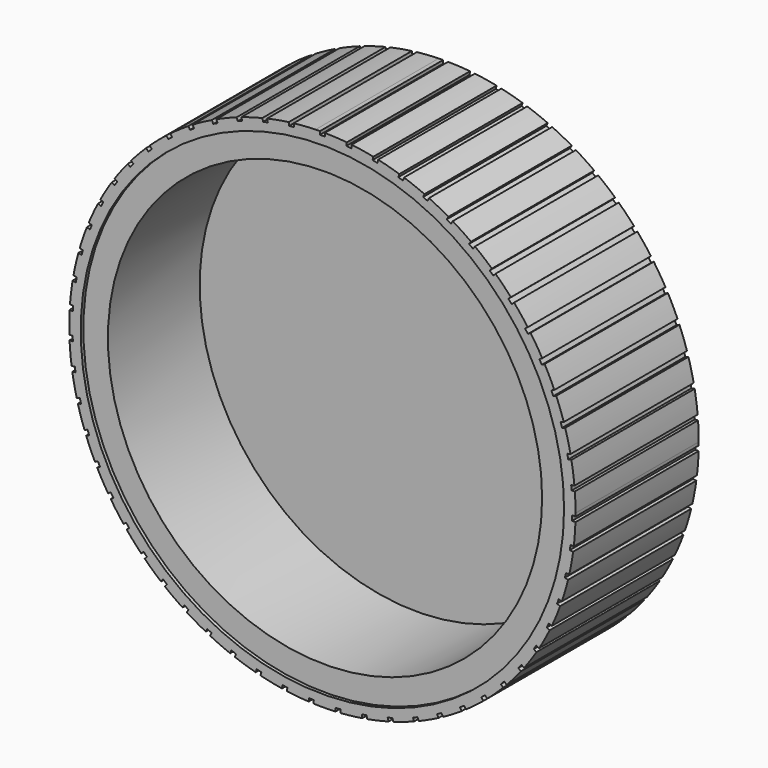
from build123d import *

# Parameters (mm, degrees)
F0_R     = 14.75
F0_R_2   = 13.25
F1_DEPTH = 9
F2_R     = 13.25
F3_DEPTH = 2
F4_R     = 14.75
F5_DEPTH = 9.2
F6_DEPTH = 0.2


# Not quite as in the source:
# - a feature names something its author has since deleted; it is built from what else it names


with BuildPart() as f1:
    # F0 (on Front) → F1 (new body)
    with BuildSketch(Plane.XZ):
        Circle(F0_R)
        Circle(F0_R_2, mode=Mode.SUBTRACT)
    extrude(amount=F1_DEPTH)

    # F2 (on Front) → F3 (join)
    with BuildSketch(Plane.XZ):
        Circle(F2_R)
    extrude(amount=F3_DEPTH)

    # F4 (on Front) → F5 (join)
    with BuildSketch(Plane.XZ):
        with BuildLine():
            ThreePointArc((15.4487973261, -0.1927723482), (15.4496993286, -0.0963880499), (15.45, 0))
            ThreePointArc((15.45, 0), (15.4393387559, 0.5738630326), (15.4073697372, 1.146934079))
            Line((15.4073697372, 1.146934079), (15.2080751315, 1.1301513458))
            Line((15.2080751315, 1.1301513458), (15.1829010317, 1.4290932544))
            Line((15.1829010317, 1.4290932544), (15.3821956374, 1.4458759876))
            ThreePointArc((15.3821956374, 1.4458759876), (15.3049999381, 2.1117473558), (15.1989934484, 2.77364348))
            Line((15.1989934484, 2.77364348), (15.0026005872, 2.7358302011))
            Line((15.0026005872, 2.7358302011), (14.9458806688, 3.0304194929))
            Line((14.9458806688, 3.0304194929), (15.14227353, 3.0682327718))
            ThreePointArc((15.14227353, 3.0682327718), (14.9949308113, 3.7221700611), (14.8193609898, 4.3691005774))
            Line((14.8193609898, 4.3691005774), (14.6280827491, 4.3106828175))
            Line((14.6280827491, 4.3106828175), (14.5404561094, 4.5976001784))
            Line((14.5404561094, 4.5976001784), (14.73173435, 4.6560179383))
            ThreePointArc((14.73173435, 4.6560179383), (14.5159048106, 5.2906528452), (14.2727499076, 5.9153283995))
            Line((14.2727499076, 5.9153283995), (14.0887415342, 5.8369643867))
            Line((14.0887415342, 5.8369643867), (13.9711955149, 6.1129769468))
            Line((13.9711955149, 6.1129769468), (14.1552038884, 6.1913409597))
            ThreePointArc((14.1552038884, 6.1913409597), (13.8733194092, 6.7995226722), (13.5653191968, 7.3949046708))
            Line((13.5653191968, 7.3949046708), (13.3906540232, 7.2974773793))
            Line((13.3906540232, 7.2974773793), (13.2445130859, 7.5594751397))
            Line((13.2445130859, 7.5594751397), (13.4191782595, 7.6569024312))
            ThreePointArc((13.4191782595, 7.6569024312), (13.0744150019, 8.2317782015), (12.705039903, 8.7911581184))
            Line((12.705039903, 8.7911581184), (12.5416859865, 8.6757653199))
            Line((12.5416859865, 8.6757653199), (12.3685967887, 8.9207961947))
            Line((12.3685967887, 8.9207961947), (12.5319507053, 9.0361889932))
            ThreePointArc((12.5319507053, 9.0361889932), (12.1281933235, 9.5712813514), (11.7016053089, 10.0883563178))
            Line((11.7016053089, 10.0883563178), (11.5514032559, 9.9562982121))
            Line((11.5514032559, 9.9562982121), (11.3533160974, 10.1816012916))
            Line((11.3533160974, 10.1816012916), (11.5035181504, 10.3136593973))
            ThreePointArc((11.5035181504, 10.3136593973), (11.045316021, 10.802939137), (10.5663217135, 11.2718829592))
            Line((10.5663217135, 11.2718829592), (10.4309639406, 11.1246475243))
            Line((10.4309639406, 11.1246475243), (10.2101107881, 11.3276841836))
            Line((10.2101107881, 11.3276841836), (10.345468561, 11.4749196186))
            ThreePointArc((10.345468561, 11.4749196186), (9.8379845219, 11.9128737317), (9.3119810375, 12.3284025387))
            Line((9.3119810375, 12.3284025387), (9.1929927019, 12.1676487643))
            Line((9.1929927019, 12.1676487643), (8.9518620403, 12.3461312677))
            Line((8.9518620403, 12.3461312677), (9.0708503759, 12.5068850421))
            ThreePointArc((9.0708503759, 12.5068850421), (8.5198025541, 12.8885788371), (7.9527166893, 13.2460106167))
            Line((7.9527166893, 13.2460106167), (7.8514385039, 13.0735498121))
            Line((7.8514385039, 13.0735498121), (7.5927472969, 13.2254670902))
            Line((7.5927472969, 13.2254670902), (7.6940254823, 13.3979278949))
            ThreePointArc((7.6940254823, 13.3979278949), (7.1056228638, 13.7190605989), (6.5038443151, 14.0143679531))
            Line((6.5038443151, 14.0143679531), (6.4214174419, 13.8321433374))
            Line((6.4214174419, 13.8321433374), (6.1480805183, 13.9557836473))
            Line((6.1480805183, 13.9557836473), (6.2305073916, 14.138008263))
            ThreePointArc((6.2305073916, 14.138008263), (5.6113798614, 14.3949614814), (4.9816892284, 14.6248170051))
            Line((4.9816892284, 14.6248170051), (4.9190424203, 14.4348818123))
            Line((4.9190424203, 14.4348818123), (4.6341396312, 14.5288520244))
            Line((4.6341396312, 14.5288520244), (4.6967864393, 14.7187872172))
            ThreePointArc((4.6967864393, 14.7187872172), (4.0539100785, 14.9086657041), (3.4034024629, 15.0704794773))
            Line((3.4034024629, 15.0704794773), (3.3612415992, 14.8749738212))
            Line((3.3612415992, 14.8749738212), (3.067983115, 14.9382151168))
            Line((3.067983115, 14.9382151168), (3.1101439788, 15.1337207729))
            ThreePointArc((3.1101439788, 15.1337207729), (2.4507624606, 15.2543850535), (1.7867675218, 15.3463338235))
            Line((1.7867675218, 15.3463338235), (1.7655676541, 15.1474605835))
            Line((1.7655676541, 15.1474605835), (1.4672577941, 15.179260385))
            Line((1.4672577941, 15.179260385), (1.4884576617, 15.378133625))
            ThreePointArc((1.4884576617, 15.378133625), (0.8200006331, 15.4282241027), (0.15, 15.4492718275))
            Line((0.15, 15.4492718275), (0.15, 15.2492718275))
            Line((0.15, 15.2492718275), (-0.1330783791, 15.2492718275))
            Line((-0.1330783791, 15.2492718275), (-0.4161136441, 15.2443314286))
            Line((-0.4161136441, 15.2443314286), (-0.4196041254, 15.4443009676))
            ThreePointArc((-0.4196041254, 15.4443009676), (-1.0891353807, 15.4115633251), (-1.7566164007, 15.3498142927))
            Line((-1.7566164007, 15.3498142927), (-1.7319489452, 15.1513413307))
            Line((-1.7319489452, 15.1513413307), (-2.0296583882, 15.1143401476))
            Line((-2.0296583882, 15.1143401476), (-2.0543258437, 15.3128131095))
            ThreePointArc((-2.0543258437, 15.3128131095), (-2.7166149255, 15.2092900343), (-3.3737901346, 15.0771363371))
            Line((-3.3737901346, 15.0771363371), (-3.328223648, 14.882396266))
            Line((-3.328223648, 14.882396266), (-3.6203337547, 14.8140465361))
            Line((-3.6203337547, 14.8140465361), (-3.6659002413, 15.0087866072))
            ThreePointArc((-3.6659002413, 15.0087866072), (-4.3134847416, 14.8356445557), (-4.9529493527, 14.6345752487))
            Line((-4.9529493527, 14.6345752487), (-4.8869972599, 14.4457623216))
            Line((-4.8869972599, 14.4457623216), (-5.1702166506, 14.3468341823))
            Line((-5.1702166506, 14.3468341823), (-5.2361687434, 14.5356471094))
            ThreePointArc((-5.2361687434, 14.5356471094), (-5.8617519395, 14.294836977), (-6.4763007215, 14.0271176285))
            Line((-6.4763007215, 14.0271176285), (-6.3907061442, 13.8463593138))
            Line((-6.3907061442, 13.8463593138), (-6.6618436163, 13.7179674479))
            Line((-6.6618436163, 13.7179674479), (-6.7474381936, 13.8987257626))
            ThreePointArc((-6.7474381936, 13.8987257626), (-7.3439712645, 13.5929609014), (-7.926679728, 13.2616080657))
            Line((-7.926679728, 13.2616080657), (-7.8224071117, 13.0909410757))
            Line((-7.8224071117, 13.0909410757), (-8.0784075967, 12.9345321512))
            Line((-8.0784075967, 12.9345321512), (-8.182680213, 13.1051991412))
            ThreePointArc((-8.182680213, 13.1051991412), (-8.7434416631, 12.7379247872), (-9.2877440825, 12.3466720155))
            Line((-9.2877440825, 12.3466720155), (-9.1659683292, 12.1880193575))
            Line((-9.1659683292, 12.1880193575), (-9.4039473162, 12.0053557275))
            Line((-9.4039473162, 12.0053557275), (-9.5257230696, 12.1640083855))
            ThreePointArc((-9.5257230696, 12.1640083855), (-10.0443944634, 11.7393628389), (-10.5441578571, 11.2926186106))
            Line((-10.5441578571, 11.2926186106), (-10.4062510871, 11.1477679192))
            Line((-10.4062510871, 11.1477679192), (-10.6235271243, 10.9409077643))
            Line((-10.6235271243, 10.9409077643), (-10.7614338942, 11.0857584558))
            ThreePointArc((-10.7614338942, 11.0857584558), (-11.2321710504, 10.6085264526), (-11.6817642845, 10.1113245028))
            Line((-11.6817642845, 10.1113245028), (-11.5292803763, 9.9819078975))
            Line((-11.5292803763, 9.9819078975), (-11.7234052843, 9.7531820351))
            Line((-11.7234052843, 9.7531820351), (-11.8758891925, 9.8825986404))
            ThreePointArc((-11.8758891925, 9.8825986404), (-12.2933880332, 9.3581574396), (-12.6877452714, 8.8161000407))
            Line((-12.6877452714, 8.8161000407), (-12.5224023524, 8.703575736))
            Line((-12.5224023524, 8.703575736), (-12.6911888095, 8.4555613575))
            Line((-12.6911888095, 8.4555613575), (-12.8565317284, 8.5680856622))
            ThreePointArc((-12.8565317284, 8.5680856622), (-13.216088044, 8.0023444573), (-13.5507658269, 7.4215392948))
            Line((-13.5507658269, 7.4215392948), (-13.374426915, 7.3271751695))
            Line((-13.374426915, 7.3271751695), (-13.5159731029, 7.0626668016))
            Line((-13.5159731029, 7.0626668016), (-13.6923120148, 7.1570309269))
            ThreePointArc((-13.6923120148, 7.1570309269), (-13.9898744687, 6.556364263), (-14.2611017811, 5.943355617))
            Line((-14.2611017811, 5.943355617), (-14.0757537924, 5.8682149283))
            Line((-14.0757537924, 5.8682149283), (-14.1884648255, 5.5901929453))
            Line((-14.1884648255, 5.5901929453), (-14.3738128141, 5.665333634))
            ThreePointArc((-14.3738128141, 5.665333634), (-14.6060285918, 5.0365095826), (-14.8107493529, 4.3982045888))
            Line((-14.8107493529, 4.3982045888), (-14.6184807144, 4.3431339919))
            Line((-14.6184807144, 4.3431339919), (-14.7010866098, 4.0547310341))
            Line((-14.7010866098, 4.0547310341), (-14.8933552483, 4.1098016311))
            ThreePointArc((-14.8933552483, 4.1098016311), (-15.0576078355, 3.4599055296), (-15.1935153338, 2.8034963531))
            Line((-15.1935153338, 2.8034963531), (-14.9964924514, 2.7691163613))
            Line((-14.9964924514, 2.7691163613), (-15.0480624391, 2.4735820378))
            Line((-15.0480624391, 2.4735820378), (-15.2450853214, 2.5079620296))
            ThreePointArc((-15.2450853214, 2.5079620296), (-15.3395239856, 1.844316647), (-15.4050868699, 1.1771994435))
            Line((-15.4050868699, 1.1771994435), (-15.2055297187, 1.1638974369))
            Line((-15.2055297187, 1.1638974369), (-15.2254827286, 0.86456171))
            Line((-15.2254827286, 0.86456171), (-15.4250398799, 0.8778637166))
            ThreePointArc((-15.4250398799, 0.8778637166), (-15.4486005241, 0.2079467433), (-15.443080058, -0.4623616779))
            Line((-15.443080058, -0.4623616779), (-15.2432371679, -0.4544358177))
            Line((-15.2432371679, -0.4544358177), (-15.2313483776, -0.7542001529))
            Line((-15.2313483776, -0.7542001529), (-15.4311912677, -0.7621260131))
            ThreePointArc((-15.4311912677, -0.7621260131), (-15.38360842, -1.4307662211), (-15.3070668061, -2.0967130931))
            Line((-15.3070668061, -2.0967130931), (-15.1091899267, -2.0676486715))
            Line((-15.1091899267, -2.0676486715), (-15.0655932942, -2.3644639906))
            Line((-15.0655932942, -2.3644639906), (-15.2634701736, -2.3935284122))
            ThreePointArc((-15.2634701736, -2.3935284122), (-15.1452799785, -3.0533578848), (-14.9985796569, -3.7074395851))
            Line((-14.9985796569, -3.7074395851), (-14.8048983856, -3.6575640883))
            Line((-14.8048983856, -3.6575640883), (-14.7300851404, -3.9480859951))
            Line((-14.7300851404, -3.9480859951), (-14.9237664116, -3.9979614919))
            ThreePointArc((-14.9237664116, -3.9979614919), (-14.7363005889, -4.6415455349), (-14.52109452, -5.2763921329))
            Line((-14.52109452, -5.2763921329), (-14.33379118, -5.206267538))
            Line((-14.33379118, -5.206267538), (-14.2286042877, -5.4872225481))
            Line((-14.2286042877, -5.4872225481), (-14.4159076278, -5.557347143))
            ThreePointArc((-14.4159076278, -5.557347143), (-14.1612784672, -6.1774341092), (-13.8799915069, -6.7858924077))
            Line((-13.8799915069, -6.7858924077), (-13.701176557, -6.6963088507))
            Line((-13.701176557, -6.6963088507), (-13.5668012214, -6.9645312755))
            Line((-13.5668012214, -6.9645312755), (-13.7456161713, -7.0541148326))
            ThreePointArc((-13.7456161713, -7.0541148326), (-13.4266927323, -7.6437178305), (-13.0824943093, -8.2189319651))
            Line((-13.0824943093, -8.2189319651), (-12.9141825648, -8.1108988375))
            Line((-12.9141825648, -8.1108988375), (-12.7521328734, -8.3633664543))
            Line((-12.7521328734, -8.3633664543), (-12.9204446179, -8.4713995819))
            ThreePointArc((-12.9204446179, -8.4713995819), (-12.540820402, -9.023875201), (-12.1375888063, -9.5593638893))
            Line((-12.1375888063, -9.5593638893), (-11.9816767365, -9.4340984652))
            Line((-11.9816767365, -9.4340984652), (-11.7937786003, -9.6679665699))
            Line((-11.7937786003, -9.6679665699), (-11.9496906701, -9.793231994))
            ThreePointArc((-11.9496906701, -9.793231994), (-11.5136431309, -10.3023551605), (-11.0559218146, -10.7920847305))
            Line((-11.0559218146, -10.7920847305), (-10.9141661742, -10.6509984504))
            Line((-10.9141661742, -10.6509984504), (-10.7025367541, -10.8636319109))
            Line((-10.7025367541, -10.8636319109), (-10.8442923945, -11.004718191))
            ThreePointArc((-10.8442923945, -11.004718191), (-10.356734741, -11.4647523089), (-9.8496811245, -11.9032046838))
            Line((-9.8496811245, -11.9032046838), (-9.7236791594, -11.7478872515))
            Line((-9.7236791594, -11.7478872515), (-9.4907030109, -11.9368901992))
            Line((-9.4907030109, -11.9368901992), (-9.616704976, -12.0922076315))
            ThreePointArc((-9.616704976, -12.0922076315), (-9.0831308126, -12.4979692207), (-8.532458173, -12.8802040949))
            Line((-8.532458173, -12.8802040949), (-8.4236296228, -12.7124055649))
            Line((-8.4236296228, -12.7124055649), (-8.1719318279, -12.8756483903))
            Line((-8.1719318279, -12.8756483903), (-8.2807603781, -13.0434469202))
            ThreePointArc((-8.2807603781, -13.0434469202), (-7.7071818047, -13.3903640216), (-7.1190949007, -13.7120745256))
            Line((-7.1190949007, -13.7120745256), (-7.0286660018, -13.5336855846))
            Line((-7.0286660018, -13.5336855846), (-6.7610825904, -13.6693289329))
            Line((-6.7610825904, -13.6693289329), (-6.8515114892, -13.8477178738))
            ThreePointArc((-6.8515114892, -13.8477178738), (-6.2443913594, -14.1318815644), (-5.6255165187, -14.3894427932))
            Line((-5.6255165187, -14.3894427932), (-5.5545061879, -14.2024734563))
            Line((-5.5545061879, -14.2024734563), (-5.2740521826, -14.3089889526))
            Line((-5.2740521826, -14.3089889526), (-5.3450625134, -14.4959582894))
            ThreePointArc((-5.3450625134, -14.4959582894), (-4.7112416136, -14.7141667266), (-4.0685520699, -14.9046765834))
            Line((-4.0685520699, -14.9046765834), (-4.0177604231, -14.7112335462))
            Line((-4.0177604231, -14.7112335462), (-3.7275958674, -14.7874210165))
            Line((-3.7275958674, -14.7874210165), (-3.7783875142, -14.9808640536))
            ThreePointArc((-3.7783875142, -14.9808640536), (-3.1250074845, -15.1306585522), (-2.4657448062, -15.2519704481))
            Line((-2.4657448062, -15.2519704481), (-2.4357441433, -15.0542333494))
            Line((-2.4357441433, -15.0542333494), (-2.1391384952, -15.0992343438))
            Line((-2.1391384952, -15.0992343438), (-2.1691391581, -15.2969714425))
            ThreePointArc((-2.1691391581, -15.2969714425), (-1.5035620228, -15.376664178), (-0.8351545177, -15.4274112194))
            Line((-0.8351545177, -15.4274112194), (-0.8262828742, -15.2276080814))
            Line((-0.8262828742, -15.2276080814), (-0.5265781672, -15.2409155467))
            Line((-0.5265781672, -15.2409155467), (-0.5354498108, -15.4407186847))
            ThreePointArc((-0.5354498108, -15.4407186847), (0.1348249734, -15.4494117113), (0.8048459573, -15.4290221007))
            Line((0.8048459573, -15.4290221007), (0.7924886194, -15.2294042253))
            Line((0.7924886194, -15.2294042253), (1.0919154326, -15.2108682184))
            Line((1.0919154326, -15.2108682184), (1.1042727705, -15.4104860938))
            ThreePointArc((1.1042727705, -15.4104860938), (1.7716928159, -15.3480814621), (2.4357777506, -15.2567849415))
            Line((2.4357777506, -15.2567849415), (2.4023306687, -15.0596015428))
            Line((2.4023306687, -15.0596015428), (2.6981057667, -15.00943092))
            Line((2.6981057667, -15.00943092), (2.7315528486, -15.2066143186))
            ThreePointArc((2.7315528486, -15.2066143186), (3.3885979334, -15.0738151788), (4.0392641758, -14.9126404409))
            Line((4.0392641758, -14.9126404409), (3.9851042182, -14.7201133025))
            Line((3.9851042182, -14.7201133025), (4.2738949258, -14.6388733662))
            Line((4.2738949258, -14.6388733662), (4.3280548833, -14.8314005046))
            ThreePointArc((4.3280548833, -14.8314005046), (4.9673216868, -14.6297031843), (5.5972377903, -14.4004662813))
            Line((5.5972377903, -14.4004662813), (5.5229752098, -14.214764722))
            Line((5.5229752098, -14.214764722), (5.8015275488, -14.1033708513))
            Line((5.8015275488, -14.1033708513), (5.8757901293, -14.2890724106))
            ThreePointArc((5.8757901293, -14.2890724106), (6.4900756491, -14.0207495544), (7.0921439714, -13.7260334361))
            Line((7.0921439714, -13.7260334361), (6.998615529, -13.5492498665))
            Line((6.998615529, -13.5492498665), (7.2637908834, -13.408957203))
            Line((7.2637908834, -13.408957203), (7.3573193258, -13.5857407726))
            ThreePointArc((7.3573193258, -13.5857407726), (7.9397020388, -13.2538157349), (8.5071387152, -12.8969411443))
            Line((8.5071387152, -12.8969411443), (8.3953982519, -12.731067491))
            Line((8.3953982519, -12.731067491), (8.6442087319, -12.5634567961))
            Line((8.6442087319, -12.5634567961), (8.7559491952, -12.7293304495))
            ThreePointArc((8.7559491952, -12.7293304495), (9.2998670463, -12.3375432288), (9.8262784276, -11.9225312859))
            Line((9.8262784276, -11.9225312859), (9.6975849902, -11.7694365467))
            Line((9.6975849902, -11.7694365467), (9.9272270991, -11.5763963906))
            Line((9.9272270991, -11.5763963906), (10.0559205364, -11.7294911298))
            ThreePointArc((10.0559205364, -11.7294911298), (10.5552448771, -11.2822562275), (11.0346995708, -10.8137831207))
            Line((11.0346995708, -10.8137831207), (10.8905032254, -10.6751923058))
            Line((10.8905032254, -10.6751923058), (11.0983894478, -10.4588977877))
            Line((11.0983894478, -10.4588977877), (11.2425857932, -10.5974886026))
            ThreePointArc((11.2425857932, -10.5974886026), (11.6916904368, -10.0998452825), (12.1187861394, -9.583189579))
            Line((12.1187861394, -9.583189579), (11.9607116327, -9.4606642742))
            Line((11.9607116327, -9.4606642742), (12.1444995899, -9.2235525141))
            Line((12.1444995899, -9.2235525141), (12.3025740966, -9.3460778189))
            ThreePointArc((12.3025740966, -9.3460778189), (12.696398712, -8.8036333264), (13.0663230802, -8.2446164958))
            Line((13.0663230802, -8.2446164958), (12.8961515323, -8.1395372672))
            Line((12.8961515323, -8.1395372672), (13.0537703753, -7.8842799454))
            Line((13.0537703753, -7.8842799454), (13.2239419232, -7.989359174))
            ThreePointArc((13.2239419232, -7.989359174), (13.5580490523, -7.4082255565), (13.8666339265, -6.8131463765))
            Line((13.8666339265, -6.8131463765), (13.6862827623, -6.7266972147))
            Line((13.6862827623, -6.7266972147), (13.8159565051, -6.4561704685))
            Line((13.8159565051, -6.4561704685), (13.9963076693, -6.5426196303))
            ThreePointArc((13.9963076693, -6.5426196303), (14.2669327267, -5.9293448686), (14.5107010963, -5.304908453))
            Line((14.5107010963, -5.304908453), (14.3222024405, -5.2380634325))
            Line((14.3222024405, -5.2380634325), (14.4224699713, -4.9553154488))
            Line((14.4224699713, -4.9553154488), (14.610968627, -5.0221604693))
            ThreePointArc((14.610968627, -5.0221604693), (14.8150623182, -4.3836546978), (14.9912674986, -3.736896946))
            Line((14.9912674986, -3.736896946), (14.7967452786, -3.6904092498))
            Line((14.7967452786, -3.6904092498), (14.8664768229, -3.3986259197))
            Line((14.8664768229, -3.3986259197), (15.060999043, -3.4451136159))
            ThreePointArc((15.060999043, -3.4451136159), (15.1962617218, -2.7885712618), (15.3029183038, -2.1267795811))
            Line((15.3029183038, -2.1267795811), (15.1045643179, -2.1011730138))
            Line((15.1045643179, -2.1011730138), (15.1429741688, -1.803642035))
            Line((15.1429741688, -1.803642035), (15.3413281547, -1.8292486023))
            ThreePointArc((15.3413281547, -1.8292486023), (15.4062357356, -1.1620673218), (15.4421419555, -0.4926985158))
            Line((15.4421419555, -0.4926985158), (15.242191177, -0.4882616021))
            Line((15.242191177, -0.4882616021), (15.2488465476, -0.1883354344))
            Line((15.2488465476, -0.1883354344), (15.4487973261, -0.1927723482))
        make_face()
        Circle(F4_R, mode=Mode.SUBTRACT)
        Polygon((-0.4161136441, 15.2443314286), (-0.1330783791, 15.2492718275), (-0.15, 15.2492718275), (-0.15, 15.4490069251), (-0.4196041254, 15.4443009676), align=None)
    extrude(amount=F5_DEPTH)

    # F4 (on Front) → F6 (join)
    with BuildSketch(Plane.XZ):
        with BuildLine():
            ThreePointArc((15.4487973261, -0.1927723482), (15.4496993286, -0.0963880499), (15.45, 0))
            ThreePointArc((15.45, 0), (15.4393387559, 0.5738630326), (15.4073697372, 1.146934079))
            Line((15.4073697372, 1.146934079), (15.2080751315, 1.1301513458))
            Line((15.2080751315, 1.1301513458), (15.1829010317, 1.4290932544))
            Line((15.1829010317, 1.4290932544), (15.3821956374, 1.4458759876))
            ThreePointArc((15.3821956374, 1.4458759876), (15.3049999381, 2.1117473558), (15.1989934484, 2.77364348))
            Line((15.1989934484, 2.77364348), (15.0026005872, 2.7358302011))
            Line((15.0026005872, 2.7358302011), (14.9458806688, 3.0304194929))
            Line((14.9458806688, 3.0304194929), (15.14227353, 3.0682327718))
            ThreePointArc((15.14227353, 3.0682327718), (14.9949308113, 3.7221700611), (14.8193609898, 4.3691005774))
            Line((14.8193609898, 4.3691005774), (14.6280827491, 4.3106828175))
            Line((14.6280827491, 4.3106828175), (14.5404561094, 4.5976001784))
            Line((14.5404561094, 4.5976001784), (14.73173435, 4.6560179383))
            ThreePointArc((14.73173435, 4.6560179383), (14.5159048106, 5.2906528452), (14.2727499076, 5.9153283995))
            Line((14.2727499076, 5.9153283995), (14.0887415342, 5.8369643867))
            Line((14.0887415342, 5.8369643867), (13.9711955149, 6.1129769468))
            Line((13.9711955149, 6.1129769468), (14.1552038884, 6.1913409597))
            ThreePointArc((14.1552038884, 6.1913409597), (13.8733194092, 6.7995226722), (13.5653191968, 7.3949046708))
            Line((13.5653191968, 7.3949046708), (13.3906540232, 7.2974773793))
            Line((13.3906540232, 7.2974773793), (13.2445130859, 7.5594751397))
            Line((13.2445130859, 7.5594751397), (13.4191782595, 7.6569024312))
            ThreePointArc((13.4191782595, 7.6569024312), (13.0744150019, 8.2317782015), (12.705039903, 8.7911581184))
            Line((12.705039903, 8.7911581184), (12.5416859865, 8.6757653199))
            Line((12.5416859865, 8.6757653199), (12.3685967887, 8.9207961947))
            Line((12.3685967887, 8.9207961947), (12.5319507053, 9.0361889932))
            ThreePointArc((12.5319507053, 9.0361889932), (12.1281933235, 9.5712813514), (11.7016053089, 10.0883563178))
            Line((11.7016053089, 10.0883563178), (11.5514032559, 9.9562982121))
            Line((11.5514032559, 9.9562982121), (11.3533160974, 10.1816012916))
            Line((11.3533160974, 10.1816012916), (11.5035181504, 10.3136593973))
            ThreePointArc((11.5035181504, 10.3136593973), (11.045316021, 10.802939137), (10.5663217135, 11.2718829592))
            Line((10.5663217135, 11.2718829592), (10.4309639406, 11.1246475243))
            Line((10.4309639406, 11.1246475243), (10.2101107881, 11.3276841836))
            Line((10.2101107881, 11.3276841836), (10.345468561, 11.4749196186))
            ThreePointArc((10.345468561, 11.4749196186), (9.8379845219, 11.9128737317), (9.3119810375, 12.3284025387))
            Line((9.3119810375, 12.3284025387), (9.1929927019, 12.1676487643))
            Line((9.1929927019, 12.1676487643), (8.9518620403, 12.3461312677))
            Line((8.9518620403, 12.3461312677), (9.0708503759, 12.5068850421))
            ThreePointArc((9.0708503759, 12.5068850421), (8.5198025541, 12.8885788371), (7.9527166893, 13.2460106167))
            Line((7.9527166893, 13.2460106167), (7.8514385039, 13.0735498121))
            Line((7.8514385039, 13.0735498121), (7.5927472969, 13.2254670902))
            Line((7.5927472969, 13.2254670902), (7.6940254823, 13.3979278949))
            ThreePointArc((7.6940254823, 13.3979278949), (7.1056228638, 13.7190605989), (6.5038443151, 14.0143679531))
            Line((6.5038443151, 14.0143679531), (6.4214174419, 13.8321433374))
            Line((6.4214174419, 13.8321433374), (6.1480805183, 13.9557836473))
            Line((6.1480805183, 13.9557836473), (6.2305073916, 14.138008263))
            ThreePointArc((6.2305073916, 14.138008263), (5.6113798614, 14.3949614814), (4.9816892284, 14.6248170051))
            Line((4.9816892284, 14.6248170051), (4.9190424203, 14.4348818123))
            Line((4.9190424203, 14.4348818123), (4.6341396312, 14.5288520244))
            Line((4.6341396312, 14.5288520244), (4.6967864393, 14.7187872172))
            ThreePointArc((4.6967864393, 14.7187872172), (4.0539100785, 14.9086657041), (3.4034024629, 15.0704794773))
            Line((3.4034024629, 15.0704794773), (3.3612415992, 14.8749738212))
            Line((3.3612415992, 14.8749738212), (3.067983115, 14.9382151168))
            Line((3.067983115, 14.9382151168), (3.1101439788, 15.1337207729))
            ThreePointArc((3.1101439788, 15.1337207729), (2.4507624606, 15.2543850535), (1.7867675218, 15.3463338235))
            Line((1.7867675218, 15.3463338235), (1.7655676541, 15.1474605835))
            Line((1.7655676541, 15.1474605835), (1.4672577941, 15.179260385))
            Line((1.4672577941, 15.179260385), (1.4884576617, 15.378133625))
            ThreePointArc((1.4884576617, 15.378133625), (0.8200006331, 15.4282241027), (0.15, 15.4492718275))
            Line((0.15, 15.4492718275), (0.15, 15.2492718275))
            Line((0.15, 15.2492718275), (-0.1330783791, 15.2492718275))
            Line((-0.1330783791, 15.2492718275), (-0.4161136441, 15.2443314286))
            Line((-0.4161136441, 15.2443314286), (-0.4196041254, 15.4443009676))
            ThreePointArc((-0.4196041254, 15.4443009676), (-1.0891353807, 15.4115633251), (-1.7566164007, 15.3498142927))
            Line((-1.7566164007, 15.3498142927), (-1.7319489452, 15.1513413307))
            Line((-1.7319489452, 15.1513413307), (-2.0296583882, 15.1143401476))
            Line((-2.0296583882, 15.1143401476), (-2.0543258437, 15.3128131095))
            ThreePointArc((-2.0543258437, 15.3128131095), (-2.7166149255, 15.2092900343), (-3.3737901346, 15.0771363371))
            Line((-3.3737901346, 15.0771363371), (-3.328223648, 14.882396266))
            Line((-3.328223648, 14.882396266), (-3.6203337547, 14.8140465361))
            Line((-3.6203337547, 14.8140465361), (-3.6659002413, 15.0087866072))
            ThreePointArc((-3.6659002413, 15.0087866072), (-4.3134847416, 14.8356445557), (-4.9529493527, 14.6345752487))
            Line((-4.9529493527, 14.6345752487), (-4.8869972599, 14.4457623216))
            Line((-4.8869972599, 14.4457623216), (-5.1702166506, 14.3468341823))
            Line((-5.1702166506, 14.3468341823), (-5.2361687434, 14.5356471094))
            ThreePointArc((-5.2361687434, 14.5356471094), (-5.8617519395, 14.294836977), (-6.4763007215, 14.0271176285))
            Line((-6.4763007215, 14.0271176285), (-6.3907061442, 13.8463593138))
            Line((-6.3907061442, 13.8463593138), (-6.6618436163, 13.7179674479))
            Line((-6.6618436163, 13.7179674479), (-6.7474381936, 13.8987257626))
            ThreePointArc((-6.7474381936, 13.8987257626), (-7.3439712645, 13.5929609014), (-7.926679728, 13.2616080657))
            Line((-7.926679728, 13.2616080657), (-7.8224071117, 13.0909410757))
            Line((-7.8224071117, 13.0909410757), (-8.0784075967, 12.9345321512))
            Line((-8.0784075967, 12.9345321512), (-8.182680213, 13.1051991412))
            ThreePointArc((-8.182680213, 13.1051991412), (-8.7434416631, 12.7379247872), (-9.2877440825, 12.3466720155))
            Line((-9.2877440825, 12.3466720155), (-9.1659683292, 12.1880193575))
            Line((-9.1659683292, 12.1880193575), (-9.4039473162, 12.0053557275))
            Line((-9.4039473162, 12.0053557275), (-9.5257230696, 12.1640083855))
            ThreePointArc((-9.5257230696, 12.1640083855), (-10.0443944634, 11.7393628389), (-10.5441578571, 11.2926186106))
            Line((-10.5441578571, 11.2926186106), (-10.4062510871, 11.1477679192))
            Line((-10.4062510871, 11.1477679192), (-10.6235271243, 10.9409077643))
            Line((-10.6235271243, 10.9409077643), (-10.7614338942, 11.0857584558))
            ThreePointArc((-10.7614338942, 11.0857584558), (-11.2321710504, 10.6085264526), (-11.6817642845, 10.1113245028))
            Line((-11.6817642845, 10.1113245028), (-11.5292803763, 9.9819078975))
            Line((-11.5292803763, 9.9819078975), (-11.7234052843, 9.7531820351))
            Line((-11.7234052843, 9.7531820351), (-11.8758891925, 9.8825986404))
            ThreePointArc((-11.8758891925, 9.8825986404), (-12.2933880332, 9.3581574396), (-12.6877452714, 8.8161000407))
            Line((-12.6877452714, 8.8161000407), (-12.5224023524, 8.703575736))
            Line((-12.5224023524, 8.703575736), (-12.6911888095, 8.4555613575))
            Line((-12.6911888095, 8.4555613575), (-12.8565317284, 8.5680856622))
            ThreePointArc((-12.8565317284, 8.5680856622), (-13.216088044, 8.0023444573), (-13.5507658269, 7.4215392948))
            Line((-13.5507658269, 7.4215392948), (-13.374426915, 7.3271751695))
            Line((-13.374426915, 7.3271751695), (-13.5159731029, 7.0626668016))
            Line((-13.5159731029, 7.0626668016), (-13.6923120148, 7.1570309269))
            ThreePointArc((-13.6923120148, 7.1570309269), (-13.9898744687, 6.556364263), (-14.2611017811, 5.943355617))
            Line((-14.2611017811, 5.943355617), (-14.0757537924, 5.8682149283))
            Line((-14.0757537924, 5.8682149283), (-14.1884648255, 5.5901929453))
            Line((-14.1884648255, 5.5901929453), (-14.3738128141, 5.665333634))
            ThreePointArc((-14.3738128141, 5.665333634), (-14.6060285918, 5.0365095826), (-14.8107493529, 4.3982045888))
            Line((-14.8107493529, 4.3982045888), (-14.6184807144, 4.3431339919))
            Line((-14.6184807144, 4.3431339919), (-14.7010866098, 4.0547310341))
            Line((-14.7010866098, 4.0547310341), (-14.8933552483, 4.1098016311))
            ThreePointArc((-14.8933552483, 4.1098016311), (-15.0576078355, 3.4599055296), (-15.1935153338, 2.8034963531))
            Line((-15.1935153338, 2.8034963531), (-14.9964924514, 2.7691163613))
            Line((-14.9964924514, 2.7691163613), (-15.0480624391, 2.4735820378))
            Line((-15.0480624391, 2.4735820378), (-15.2450853214, 2.5079620296))
            ThreePointArc((-15.2450853214, 2.5079620296), (-15.3395239856, 1.844316647), (-15.4050868699, 1.1771994435))
            Line((-15.4050868699, 1.1771994435), (-15.2055297187, 1.1638974369))
            Line((-15.2055297187, 1.1638974369), (-15.2254827286, 0.86456171))
            Line((-15.2254827286, 0.86456171), (-15.4250398799, 0.8778637166))
            ThreePointArc((-15.4250398799, 0.8778637166), (-15.4486005241, 0.2079467433), (-15.443080058, -0.4623616779))
            Line((-15.443080058, -0.4623616779), (-15.2432371679, -0.4544358177))
            Line((-15.2432371679, -0.4544358177), (-15.2313483776, -0.7542001529))
            Line((-15.2313483776, -0.7542001529), (-15.4311912677, -0.7621260131))
            ThreePointArc((-15.4311912677, -0.7621260131), (-15.38360842, -1.4307662211), (-15.3070668061, -2.0967130931))
            Line((-15.3070668061, -2.0967130931), (-15.1091899267, -2.0676486715))
            Line((-15.1091899267, -2.0676486715), (-15.0655932942, -2.3644639906))
            Line((-15.0655932942, -2.3644639906), (-15.2634701736, -2.3935284122))
            ThreePointArc((-15.2634701736, -2.3935284122), (-15.1452799785, -3.0533578848), (-14.9985796569, -3.7074395851))
            Line((-14.9985796569, -3.7074395851), (-14.8048983856, -3.6575640883))
            Line((-14.8048983856, -3.6575640883), (-14.7300851404, -3.9480859951))
            Line((-14.7300851404, -3.9480859951), (-14.9237664116, -3.9979614919))
            ThreePointArc((-14.9237664116, -3.9979614919), (-14.7363005889, -4.6415455349), (-14.52109452, -5.2763921329))
            Line((-14.52109452, -5.2763921329), (-14.33379118, -5.206267538))
            Line((-14.33379118, -5.206267538), (-14.2286042877, -5.4872225481))
            Line((-14.2286042877, -5.4872225481), (-14.4159076278, -5.557347143))
            ThreePointArc((-14.4159076278, -5.557347143), (-14.1612784672, -6.1774341092), (-13.8799915069, -6.7858924077))
            Line((-13.8799915069, -6.7858924077), (-13.701176557, -6.6963088507))
            Line((-13.701176557, -6.6963088507), (-13.5668012214, -6.9645312755))
            Line((-13.5668012214, -6.9645312755), (-13.7456161713, -7.0541148326))
            ThreePointArc((-13.7456161713, -7.0541148326), (-13.4266927323, -7.6437178305), (-13.0824943093, -8.2189319651))
            Line((-13.0824943093, -8.2189319651), (-12.9141825648, -8.1108988375))
            Line((-12.9141825648, -8.1108988375), (-12.7521328734, -8.3633664543))
            Line((-12.7521328734, -8.3633664543), (-12.9204446179, -8.4713995819))
            ThreePointArc((-12.9204446179, -8.4713995819), (-12.540820402, -9.023875201), (-12.1375888063, -9.5593638893))
            Line((-12.1375888063, -9.5593638893), (-11.9816767365, -9.4340984652))
            Line((-11.9816767365, -9.4340984652), (-11.7937786003, -9.6679665699))
            Line((-11.7937786003, -9.6679665699), (-11.9496906701, -9.793231994))
            ThreePointArc((-11.9496906701, -9.793231994), (-11.5136431309, -10.3023551605), (-11.0559218146, -10.7920847305))
            Line((-11.0559218146, -10.7920847305), (-10.9141661742, -10.6509984504))
            Line((-10.9141661742, -10.6509984504), (-10.7025367541, -10.8636319109))
            Line((-10.7025367541, -10.8636319109), (-10.8442923945, -11.004718191))
            ThreePointArc((-10.8442923945, -11.004718191), (-10.356734741, -11.4647523089), (-9.8496811245, -11.9032046838))
            Line((-9.8496811245, -11.9032046838), (-9.7236791594, -11.7478872515))
            Line((-9.7236791594, -11.7478872515), (-9.4907030109, -11.9368901992))
            Line((-9.4907030109, -11.9368901992), (-9.616704976, -12.0922076315))
            ThreePointArc((-9.616704976, -12.0922076315), (-9.0831308126, -12.4979692207), (-8.532458173, -12.8802040949))
            Line((-8.532458173, -12.8802040949), (-8.4236296228, -12.7124055649))
            Line((-8.4236296228, -12.7124055649), (-8.1719318279, -12.8756483903))
            Line((-8.1719318279, -12.8756483903), (-8.2807603781, -13.0434469202))
            ThreePointArc((-8.2807603781, -13.0434469202), (-7.7071818047, -13.3903640216), (-7.1190949007, -13.7120745256))
            Line((-7.1190949007, -13.7120745256), (-7.0286660018, -13.5336855846))
            Line((-7.0286660018, -13.5336855846), (-6.7610825904, -13.6693289329))
            Line((-6.7610825904, -13.6693289329), (-6.8515114892, -13.8477178738))
            ThreePointArc((-6.8515114892, -13.8477178738), (-6.2443913594, -14.1318815644), (-5.6255165187, -14.3894427932))
            Line((-5.6255165187, -14.3894427932), (-5.5545061879, -14.2024734563))
            Line((-5.5545061879, -14.2024734563), (-5.2740521826, -14.3089889526))
            Line((-5.2740521826, -14.3089889526), (-5.3450625134, -14.4959582894))
            ThreePointArc((-5.3450625134, -14.4959582894), (-4.7112416136, -14.7141667266), (-4.0685520699, -14.9046765834))
            Line((-4.0685520699, -14.9046765834), (-4.0177604231, -14.7112335462))
            Line((-4.0177604231, -14.7112335462), (-3.7275958674, -14.7874210165))
            Line((-3.7275958674, -14.7874210165), (-3.7783875142, -14.9808640536))
            ThreePointArc((-3.7783875142, -14.9808640536), (-3.1250074845, -15.1306585522), (-2.4657448062, -15.2519704481))
            Line((-2.4657448062, -15.2519704481), (-2.4357441433, -15.0542333494))
            Line((-2.4357441433, -15.0542333494), (-2.1391384952, -15.0992343438))
            Line((-2.1391384952, -15.0992343438), (-2.1691391581, -15.2969714425))
            ThreePointArc((-2.1691391581, -15.2969714425), (-1.5035620228, -15.376664178), (-0.8351545177, -15.4274112194))
            Line((-0.8351545177, -15.4274112194), (-0.8262828742, -15.2276080814))
            Line((-0.8262828742, -15.2276080814), (-0.5265781672, -15.2409155467))
            Line((-0.5265781672, -15.2409155467), (-0.5354498108, -15.4407186847))
            ThreePointArc((-0.5354498108, -15.4407186847), (0.1348249734, -15.4494117113), (0.8048459573, -15.4290221007))
            Line((0.8048459573, -15.4290221007), (0.7924886194, -15.2294042253))
            Line((0.7924886194, -15.2294042253), (1.0919154326, -15.2108682184))
            Line((1.0919154326, -15.2108682184), (1.1042727705, -15.4104860938))
            ThreePointArc((1.1042727705, -15.4104860938), (1.7716928159, -15.3480814621), (2.4357777506, -15.2567849415))
            Line((2.4357777506, -15.2567849415), (2.4023306687, -15.0596015428))
            Line((2.4023306687, -15.0596015428), (2.6981057667, -15.00943092))
            Line((2.6981057667, -15.00943092), (2.7315528486, -15.2066143186))
            ThreePointArc((2.7315528486, -15.2066143186), (3.3885979334, -15.0738151788), (4.0392641758, -14.9126404409))
            Line((4.0392641758, -14.9126404409), (3.9851042182, -14.7201133025))
            Line((3.9851042182, -14.7201133025), (4.2738949258, -14.6388733662))
            Line((4.2738949258, -14.6388733662), (4.3280548833, -14.8314005046))
            ThreePointArc((4.3280548833, -14.8314005046), (4.9673216868, -14.6297031843), (5.5972377903, -14.4004662813))
            Line((5.5972377903, -14.4004662813), (5.5229752098, -14.214764722))
            Line((5.5229752098, -14.214764722), (5.8015275488, -14.1033708513))
            Line((5.8015275488, -14.1033708513), (5.8757901293, -14.2890724106))
            ThreePointArc((5.8757901293, -14.2890724106), (6.4900756491, -14.0207495544), (7.0921439714, -13.7260334361))
            Line((7.0921439714, -13.7260334361), (6.998615529, -13.5492498665))
            Line((6.998615529, -13.5492498665), (7.2637908834, -13.408957203))
            Line((7.2637908834, -13.408957203), (7.3573193258, -13.5857407726))
            ThreePointArc((7.3573193258, -13.5857407726), (7.9397020388, -13.2538157349), (8.5071387152, -12.8969411443))
            Line((8.5071387152, -12.8969411443), (8.3953982519, -12.731067491))
            Line((8.3953982519, -12.731067491), (8.6442087319, -12.5634567961))
            Line((8.6442087319, -12.5634567961), (8.7559491952, -12.7293304495))
            ThreePointArc((8.7559491952, -12.7293304495), (9.2998670463, -12.3375432288), (9.8262784276, -11.9225312859))
            Line((9.8262784276, -11.9225312859), (9.6975849902, -11.7694365467))
            Line((9.6975849902, -11.7694365467), (9.9272270991, -11.5763963906))
            Line((9.9272270991, -11.5763963906), (10.0559205364, -11.7294911298))
            ThreePointArc((10.0559205364, -11.7294911298), (10.5552448771, -11.2822562275), (11.0346995708, -10.8137831207))
            Line((11.0346995708, -10.8137831207), (10.8905032254, -10.6751923058))
            Line((10.8905032254, -10.6751923058), (11.0983894478, -10.4588977877))
            Line((11.0983894478, -10.4588977877), (11.2425857932, -10.5974886026))
            ThreePointArc((11.2425857932, -10.5974886026), (11.6916904368, -10.0998452825), (12.1187861394, -9.583189579))
            Line((12.1187861394, -9.583189579), (11.9607116327, -9.4606642742))
            Line((11.9607116327, -9.4606642742), (12.1444995899, -9.2235525141))
            Line((12.1444995899, -9.2235525141), (12.3025740966, -9.3460778189))
            ThreePointArc((12.3025740966, -9.3460778189), (12.696398712, -8.8036333264), (13.0663230802, -8.2446164958))
            Line((13.0663230802, -8.2446164958), (12.8961515323, -8.1395372672))
            Line((12.8961515323, -8.1395372672), (13.0537703753, -7.8842799454))
            Line((13.0537703753, -7.8842799454), (13.2239419232, -7.989359174))
            ThreePointArc((13.2239419232, -7.989359174), (13.5580490523, -7.4082255565), (13.8666339265, -6.8131463765))
            Line((13.8666339265, -6.8131463765), (13.6862827623, -6.7266972147))
            Line((13.6862827623, -6.7266972147), (13.8159565051, -6.4561704685))
            Line((13.8159565051, -6.4561704685), (13.9963076693, -6.5426196303))
            ThreePointArc((13.9963076693, -6.5426196303), (14.2669327267, -5.9293448686), (14.5107010963, -5.304908453))
            Line((14.5107010963, -5.304908453), (14.3222024405, -5.2380634325))
            Line((14.3222024405, -5.2380634325), (14.4224699713, -4.9553154488))
            Line((14.4224699713, -4.9553154488), (14.610968627, -5.0221604693))
            ThreePointArc((14.610968627, -5.0221604693), (14.8150623182, -4.3836546978), (14.9912674986, -3.736896946))
            Line((14.9912674986, -3.736896946), (14.7967452786, -3.6904092498))
            Line((14.7967452786, -3.6904092498), (14.8664768229, -3.3986259197))
            Line((14.8664768229, -3.3986259197), (15.060999043, -3.4451136159))
            ThreePointArc((15.060999043, -3.4451136159), (15.1962617218, -2.7885712618), (15.3029183038, -2.1267795811))
            Line((15.3029183038, -2.1267795811), (15.1045643179, -2.1011730138))
            Line((15.1045643179, -2.1011730138), (15.1429741688, -1.803642035))
            Line((15.1429741688, -1.803642035), (15.3413281547, -1.8292486023))
            ThreePointArc((15.3413281547, -1.8292486023), (15.4062357356, -1.1620673218), (15.4421419555, -0.4926985158))
            Line((15.4421419555, -0.4926985158), (15.242191177, -0.4882616021))
            Line((15.242191177, -0.4882616021), (15.2488465476, -0.1883354344))
            Line((15.2488465476, -0.1883354344), (15.4487973261, -0.1927723482))
        make_face()
        Circle(F4_R, mode=Mode.SUBTRACT)
        Polygon((-0.4161136441, 15.2443314286), (-0.1330783791, 15.2492718275), (-0.15, 15.2492718275), (-0.15, 15.4490069251), (-0.4196041254, 15.4443009676), align=None)
    extrude(amount=-F6_DEPTH)


solid = f1.part
